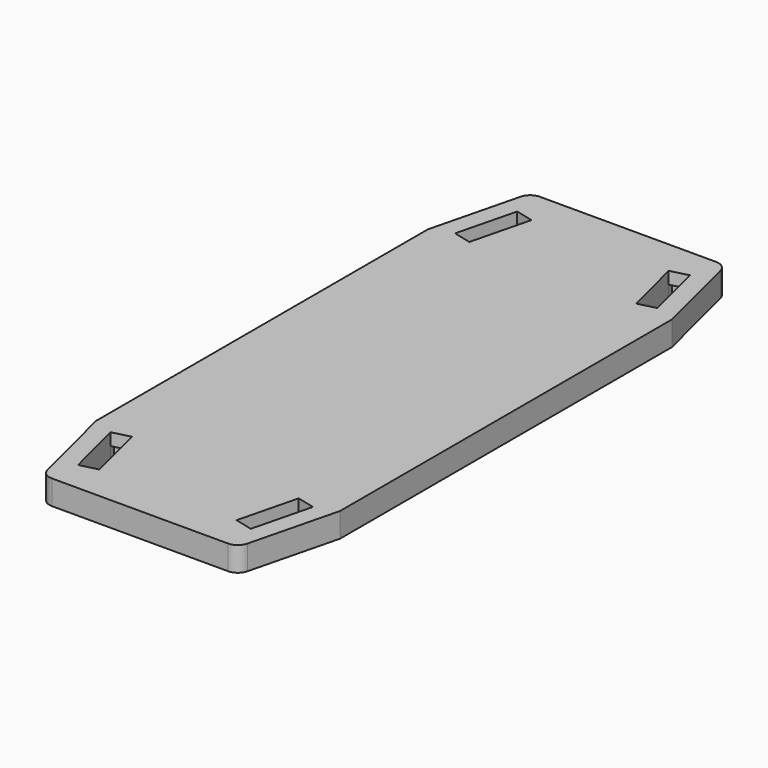
from build123d import *

# Parameters (mm, degrees)
F0_W         = 20
F0_H         = 50
F1_DEPTH     = 2
F2_SIZE2     = 2
F2_SIZE      = 8
F2_2_SIZE2   = 2
F2_2_SIZE    = 8
F3_SIZE2     = 8
F3_SIZE      = 2
F4_R         = 1
F6_DEPTH     = 2.001
F5_TEXT_SIZE = 9.7222222222
F7_DEPTH     = 1
F8_DEPTH     = 1


# Not quite as in the source:
# - a feature names something its author has since deleted; it is built from what else it names
# - Text() gives the source's letters only with a copy of the font that has no kerning and outlines rounded to 1/6400 em; it was checked with that copy


with BuildPart() as f1:
    # F0 (on Top) → F1 (new body)
    with BuildSketch(Plane.XY):
        Rectangle(F0_W, F0_H)
    extrude(amount=-F1_DEPTH)

    # F2
    f2_edges = [f1.edges().sort_by_distance(p)[0] for p in [
        (-10, 25, -1),
    ]]
    f2_side = f1.faces().sort_by_distance((-10, 0, -1))[0]
    chamfer(f2_edges, length=F2_SIZE, length2=F2_SIZE2, reference=f2_side)

    # F2#2
    f2_2_edges = [f1.edges().sort_by_distance(p)[0] for p in [
        (10, 25, -1),
    ]]
    f2_2_side = f1.faces().sort_by_distance((10, 0, -1))[0]
    chamfer(f2_2_edges, length=F2_2_SIZE, length2=F2_2_SIZE2, reference=f2_2_side)

    # F3
    f3_edges = [f1.edges().sort_by_distance(p)[0] for p in [
        (-10, -25, -1),
        (10, -25, -1),
    ]]
    f3_side = f1.faces().sort_by_distance((0, -25, -1))[0]
    chamfer(f3_edges, length=F3_SIZE, length2=F3_SIZE2, reference=f3_side)

    # F4
    f4_edges = [f1.edges().sort_by_distance(p)[0] for p in [
        (8, -25, -1),
        (-8, -25, -1),
        (-8, 25, -1),
        (8, 25, -1),
    ]]
    fillet(f4_edges, radius=F4_R)

    # F5 (on face) → F6 (cut, through all)
    with BuildSketch(Plane(origin=(0, 0, -2), x_dir=(1, 0, 0), z_dir=(0, 0, -1))):
        Polygon((-5.6236216402, 22.1361965624), (-7.0788353904, 22.5), (-8.2915135156, 17.6492874993), (-6.8362997654, 17.2854840617), align=None)
        Polygon((8.2915135156, 17.6492874993), (7.0788353904, 22.5), (5.6236216402, 22.1361965624), (6.8362997654, 17.2854840617), align=None)
        Polygon((6.8362997654, -17.2854840617), (5.6236216402, -22.1361965624), (7.0788353904, -22.5), (8.2915135156, -17.6492874993), align=None)
        Polygon((-7.0788353904, -22.5), (-5.6236216402, -22.1361965624), (-6.8362997654, -17.2854840617), (-8.2915135156, -17.6492874993), align=None)
    extrude(amount=-F6_DEPTH, mode=Mode.SUBTRACT)

    # F5 (on face) → F7 (join)
    with BuildSketch(Plane(origin=(0, 0, -2), x_dir=(1, 0, 0), z_dir=(0, 0, -1))):
        with Locations(Location((-3.5, 19.9115668403), (0, 0, -90))):
            Text('AIRSTER', F5_TEXT_SIZE, font='Open Sans', font_style=FontStyle.BOLD, text_align=(TextAlign.LEFT, TextAlign.BOTTOM))
    extrude(amount=F7_DEPTH)

    # F5 (on face) → F8 (cut)
    with BuildSketch(Plane(origin=(0, 0, -2), x_dir=(1, 0, 0), z_dir=(0, 0, -1))):
        Polygon((5.6236216402, 22.1361965624), (7.0788353904, 22.5), (6.9575675779, 22.9850712501), (5.5023538277, 22.6212678125), align=None)
        Polygon((8.4127813281, 17.1642162492), (8.2915135156, 17.6492874993), (6.8362997654, 17.2854840617), (6.9575675779, 16.8004128116), align=None)
        Polygon((-6.9575675779, 22.9850712501), (-7.0788353904, 22.5), (-5.6236216402, 22.1361965624), (-5.5023538277, 22.6212678125), align=None)
        Polygon((-6.8362997654, 17.2854840617), (-8.2915135156, 17.6492874993), (-8.4127813281, 17.1642162492), (-6.9575675779, 16.8004128116), align=None)
        Polygon((6.9575675779, -16.8004128116), (6.8362997654, -17.2854840617), (8.2915135156, -17.6492874993), (8.4127813281, -17.1642162492), align=None)
        Polygon((7.0788353904, -22.5), (5.6236216402, -22.1361965624), (5.5023538277, -22.6212678125), (6.9575675779, -22.9850712501), align=None)
        Polygon((-5.5023538277, -22.6212678125), (-5.6236216402, -22.1361965624), (-7.0788353904, -22.5), (-6.9575675779, -22.9850712501), align=None)
        Polygon((-8.2915135156, -17.6492874993), (-6.8362997654, -17.2854840617), (-6.9575675779, -16.8004128116), (-8.4127813281, -17.1642162492), align=None)
    extrude(amount=-F8_DEPTH, mode=Mode.SUBTRACT)


solid = f1.part
